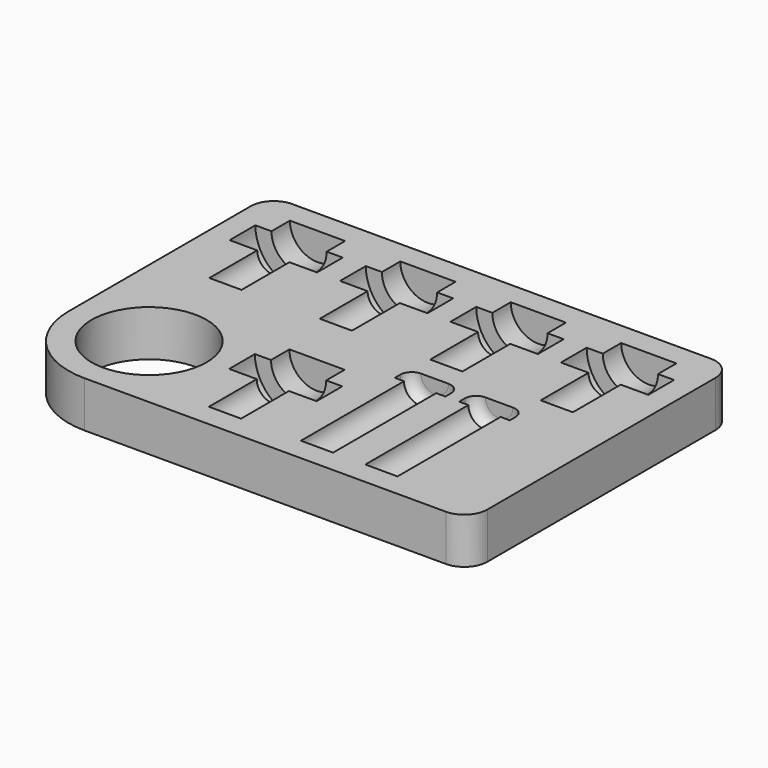
from build123d import *

# Parameters (mm, degrees)
F0_R          = 12.5
F1_DEPTH      = 10
F10_TEXT_SIZE = 5.5555555556
F11_DEPTH     = 1


# Not quite as in the source:
# - Text() gives the source's letters only with a copy of the font that has no kerning and outlines rounded to 1/6400 em; it was checked with that copy


with BuildPart() as f1:
    # F0 (on Top) → F1 (new body)
    with BuildSketch(Plane.XY):
        with BuildLine():
            ThreePointArc((0, 17.5), (5.1256313292, 5.1256313292), (17.5, 0))
            Line((17.5, 0), (96, 0))
            ThreePointArc((96, 0), (99.5355339059, 1.4644660941), (101, 5))
            Line((101, 5), (101, 67))
            ThreePointArc((101, 67), (99.5355339059, 70.5355339059), (96, 72))
            Line((96, 72), (5, 72))
            ThreePointArc((5, 72), (1.4644660941, 70.5355339059), (0, 67))
            Line((0, 67), (0, 17.5))
        make_face()
        with Locations((17.5, 17.5)):
            Circle(F0_R, mode=Mode.SUBTRACT)
    extrude(amount=F1_DEPTH)

    # F2 (on face) → F3 (revolve, cut)
    with BuildSketch(Plane.XY.offset(10)):
        Polygon((38.5, 55), (38.5, 42), (42, 42), (42, 55), (48, 55), (48, 62), (44.5, 62), (44.5, 67), (38.5, 67), (38.5, 62), align=None)
    revolve(axis=Axis((38.5, 48.5, 10), (0, 1, 0)), mode=Mode.SUBTRACT)

    # F2 (on face) → F4 (revolve, cut)
    with BuildSketch(Plane.XY.offset(10)):
        Polygon((14.5, 55), (14.5, 42), (18, 42), (18, 55), (24, 55), (24, 62), (20.5, 62), (20.5, 67), (14.5, 67), (14.5, 62), align=None)
    revolve(axis=Axis((14.5, 48.5, 10), (0, 1, 0)), mode=Mode.SUBTRACT)

    # F2 (on face) → F5 (revolve, cut)
    with BuildSketch(Plane.XY.offset(10)):
        Polygon((62.5, 55), (62.5, 42), (66, 42), (66, 55), (72, 55), (72, 62), (68.5, 62), (68.5, 67), (62.5, 67), (62.5, 62), align=None)
    revolve(axis=Axis((62.5, 48.5, 10), (0, 1, 0)), mode=Mode.SUBTRACT)

    # F2 (on face) → F6 (revolve, cut)
    with BuildSketch(Plane.XY.offset(10)):
        with BuildLine():
            Line((64, 33), (64, 5))
            Line((64, 5), (67.5, 5))
            Line((67.5, 5), (67.5, 33))
            Line((67.5, 33), (69.5, 33))
            Line((69.5, 33), (69.5, 34.5))
            ThreePointArc((69.5, 34.5), (68.767766953, 36.267766953), (67, 37))
            Line((67, 37), (64, 37))
            Line((64, 37), (64, 33))
        make_face()
    revolve(axis=Axis((64, 19, 10), (0, 1, 0)), mode=Mode.SUBTRACT)

    # F2 (on face) → F7 (revolve, cut)
    with BuildSketch(Plane.XY.offset(10)):
        with BuildLine():
            Line((78, 33), (78, 5))
            Line((78, 5), (81.5, 5))
            Line((81.5, 5), (81.5, 33))
            Line((81.5, 33), (83.5, 33))
            Line((83.5, 33), (83.5, 34.5))
            ThreePointArc((83.5, 34.5), (82.767766953, 36.267766953), (81, 37))
            Line((81, 37), (78, 37))
            Line((78, 37), (78, 33))
        make_face()
    revolve(axis=Axis((78, 19, 10), (0, 1, 0)), mode=Mode.SUBTRACT)

    # F2 (on face) → F8 (revolve, cut)
    with BuildSketch(Plane.XY.offset(10)):
        Polygon((86.5, 55), (86.5, 42), (90, 42), (90, 55), (96, 55), (96, 62), (92.5, 62), (92.5, 67), (86.5, 67), (86.5, 62), align=None)
    revolve(axis=Axis((86.5, 48.5, 10), (0, 1, 0)), mode=Mode.SUBTRACT)

    # F2 (on face) → F9 (revolve, cut)
    with BuildSketch(Plane.XY.offset(10)):
        Polygon((44, 18), (44, 5), (47.5, 5), (47.5, 18), (53.5, 18), (53.5, 25), (50, 25), (50, 30), (44, 30), (44, 25), align=None)
    revolve(axis=Axis((44, 11.5, 10), (0, 1, 0)), mode=Mode.SUBTRACT)

    # F10 (on face) → F11 (cut)
    with BuildSketch(Plane(origin=(0, 0, 0), x_dir=(1, 0, 0), z_dir=(0, 0, -1))):
        with Locations((30, -9)):
            Text('968', F10_TEXT_SIZE, font='Open Sans', text_align=(TextAlign.LEFT, TextAlign.BOTTOM))
    extrude(amount=-F11_DEPTH, mode=Mode.SUBTRACT)


solid = f1.part
